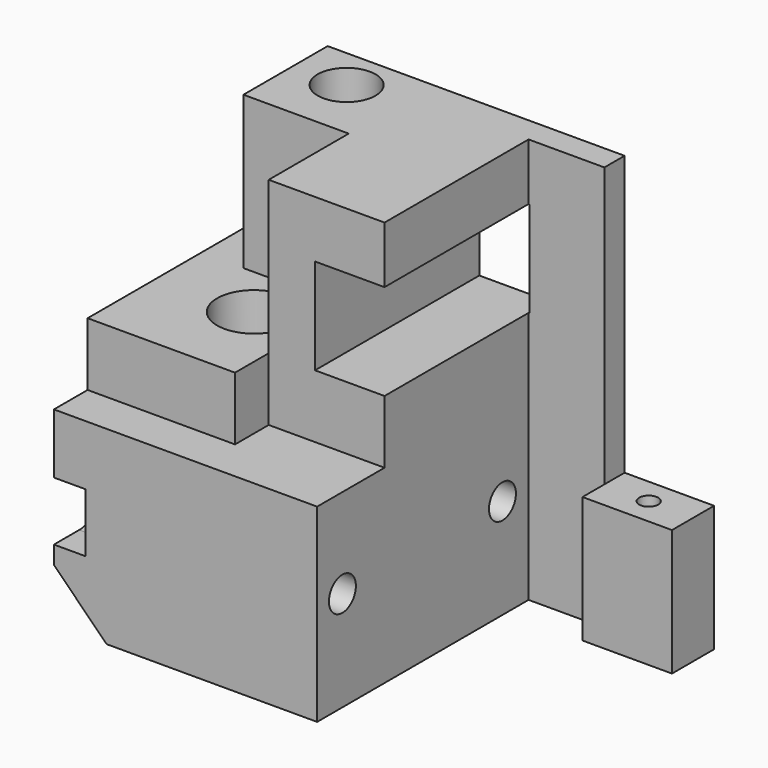
from build123d import *

# Parameters (mm, degrees)
F0_R          = 1.6
F1_DEPTH      = 16
F1_DEPTH_BACK = 9
F3_R          = 3.5
F3_R_2        = 1.4
F4_DEPTH      = 22
F5_DEPTH      = 16.501
F8_R          = 9.65
F9_DEPTH      = 5
F10_R         = 4.25
F11_DEPTH     = 6.5
F12_W         = 25
F12_H         = 9.1
F13_DEPTH     = 6.6
F14_R         = 2.8
F15_DEPTH     = 3
F16_W         = 8
F16_H         = 6
F16_H_2       = 9.1
F17_DEPTH     = 11
F23_W         = 8
F23_H         = 14.5
F24_DEPTH     = 25.001
F25_W         = 14
F25_H         = 9.5
F26_DEPTH     = 14.5
F28_DEPTH     = 9.0010001359
F29_W         = 14
F29_H         = 4
F30_DEPTH     = 6
F32_DEPTH     = 2.4
F33_W         = 10
F33_H         = 14.5
F34_DEPTH     = 4
F35_R         = 0.9
F36_DEPTH     = 3.2
F37_W         = 8.5
F37_H         = 12
F38_DEPTH     = 5
F39_R         = 0.9
F40_DEPTH     = 12
F41_SIZE      = 0.25
F42_T1_DEPTH  = 31.0668298797
F42_T3_DEPTH  = 28.5668298797


# Not quite as in the source:
# - a fillet or chamfer that OpenCascade refuses, or shapes differently, is made with other operations: its cross-section is extruded or revolved along the edge and cut away or added


with BuildPart() as f1:
    # F0 (on Right) → F1 (new body, two sides)
    with BuildSketch(Plane.YZ) as f1_sk:
        Polygon((-12.5, 0), (15, 0), (15, 38.5), (-10, 38.5), (-10, 24), (-12.5, 24), align=None)
        with Locations((-9.5, 9.5)):
            Circle(F0_R, mode=Mode.SUBTRACT)
        with Locations((9.5, 9.5)):
            Circle(F0_R, mode=Mode.SUBTRACT)
    extrude(amount=F1_DEPTH)
    extrude(f1_sk.sketch, amount=-F1_DEPTH_BACK)

    # F3 (on face) → F4 (cut)
    with BuildSketch(Plane(origin=(0, 0, 0), x_dir=(1, 0, 0), z_dir=(0, 0, -1))):
        Circle(F3_R)
        with Locations((-2.2609790798, 6.2119889676)):
            Circle(F3_R_2)
        with Locations((-4.2492507141, -5.0640598044)):
            Circle(F3_R_2)
        with Locations((6.5102297939, -1.1479291633)):
            Circle(F3_R_2)
    extrude(amount=-F4_DEPTH, mode=Mode.SUBTRACT)

    # F5 (cut, through all): a face of the model
    f5_faces = [f1.faces().sort_by_distance(p)[0] for p in [
        (0, 0, 22),
    ]]
    extrude(f5_faces, amount=-F5_DEPTH, mode=Mode.SUBTRACT)

    # F8 (on face) → F9 (cut)
    with BuildSketch(Plane(origin=(0, 0, 0), x_dir=(1, 0, 0), z_dir=(0, 0, -1))):
        Circle(F8_R)
    extrude(amount=-F9_DEPTH, mode=Mode.SUBTRACT)

    # F10 (on face) → F11 (cut)
    with BuildSketch(Plane(origin=(0, 0, 5), x_dir=(1, 0, 0), z_dir=(0, 0, -1))):
        Circle(F10_R)
    extrude(amount=-F11_DEPTH, mode=Mode.SUBTRACT)

    # F12 (on face) → F13 (cut)
    with BuildSketch(Plane.YZ.offset(16)):
        with Locations((2.5, 28.55)):
            Rectangle(F12_W, F12_H)
    extrude(amount=-F13_DEPTH, mode=Mode.SUBTRACT)

    # F14 (on face) → F15 (cut)
    with BuildSketch(Plane(origin=(-9, 0, 0), x_dir=(0, -1, 0), z_dir=(-1, 0, 0))):
        with Locations((-9.5, 9.5)):
            Circle(F14_R)
        with BuildLine():
            ThreePointArc((9.5, 6.7), (11.4798989873, 7.5201010127), (12.3, 9.5))
            ThreePointArc((12.3, 9.5), (11.4798989873, 11.4798989873), (9.5, 12.3))
            ThreePointArc((9.5, 12.3), (6.7, 9.5), (9.5, 6.7))
        make_face()
        with BuildLine():
            ThreePointArc((9.5, 12.3), (11.4798989873, 11.4798989873), (12.3, 9.5))
            ThreePointArc((12.3, 9.5), (11.4798989873, 7.5201010127), (9.5, 6.7))
            Line((9.5, 6.7), (12.5, 6.7))
            Line((12.5, 6.7), (12.5, 12.3))
            Line((12.5, 12.3), (9.5, 12.3))
        make_face()
    extrude(amount=-F15_DEPTH, mode=Mode.SUBTRACT)

    # F16 (on face) → F17 (cut)
    with BuildSketch(Plane.YZ.offset(16)):
        with Locations((-8.5, 21)):
            Rectangle(F16_W, F16_H)
        with Locations((-8.5, 28.55)):
            Rectangle(F16_W, F16_H_2)
    extrude(amount=-F17_DEPTH, mode=Mode.SUBTRACT)

    # F21 (on plane+point) → F22 (revolve, cut)
    with BuildSketch(Plane.XZ.offset(-11)):
        Polygon((0, 12.5), (0, 38.5), (-2.75, 38.5), (-2.75, 31.8), (-1.4, 31.8), (-1.4, 12.5), align=None)
    revolve(axis=Axis((0, 11, 25.5), (0, 0, 1)), mode=Mode.SUBTRACT)

    # F23 (on face) → F24 (cut, through all)
    with BuildSketch(Plane.YZ.offset(16)):
        with Locations((-8.5, 31.25)):
            Rectangle(F23_W, F23_H)
    extrude(amount=-F24_DEPTH, mode=Mode.SUBTRACT)

    # F25 (on face) → F26 (cut, through all)
    with BuildSketch(Plane.XY.offset(38.5)):
        with Locations((-2, 0.25)):
            Rectangle(F25_W, F25_H)
    extrude(amount=-F26_DEPTH, mode=Mode.SUBTRACT)

    # F27 (on face) → F28 (cut, through all)
    with BuildSketch(Plane(origin=(-9, 0, 0), x_dir=(0, -1, 0), z_dir=(-1, 0, 0))):
        with BuildLine():
            Line((-9.65, 0), (9.65, 0))
            ThreePointArc((9.65, 0), (7.4518594557, 3.5930041952), (3.4817380717, 5))
            Line((3.4817380717, 5), (-3.4817380717, 5))
            ThreePointArc((-3.4817380717, 5), (-7.4518594557, 3.5930041952), (-9.65, 0))
        make_face()
    extrude(amount=-F28_DEPTH, mode=Mode.SUBTRACT)

    # F29 (on face) → F30 (cut, through all)
    with BuildSketch(Plane.XY.offset(24)):
        with Locations((-2, -10.5)):
            Rectangle(F29_W, F29_H)
    extrude(amount=-F30_DEPTH, mode=Mode.SUBTRACT)

    # F31 (on face) → F32 (join)
    with BuildSketch(Plane(origin=(0, 15, 0), x_dir=(-1, 0, 0), z_dir=(0, 1, 0))):
        Polygon((-23.2, 0), (-16, 0), (-16, 24), (-16.1, 24), (-16.1, 33.1), (-16, 33.1), (-16, 38.5), (-23.2, 38.5), align=None)
    extrude(amount=-F32_DEPTH)

    # F33 (on face) → F34 (cut)
    with BuildSketch(Plane(origin=(-9, 0, 0), x_dir=(0, -1, 0), z_dir=(-1, 0, 0))):
        with Locations((-10, 31.25)):
            Rectangle(F33_W, F33_H)
    extrude(amount=-F34_DEPTH, mode=Mode.SUBTRACT)

    # F35 (on face) → F36 (cut)
    with BuildSketch(Plane(origin=(-5, 0, 0), x_dir=(0, -1, 0), z_dir=(-1, 0, 0))):
        with Locations((-10, 33.75)):
            Circle(F35_R)
        with Locations((-10, 27.25)):
            Circle(F35_R)
    extrude(amount=-F36_DEPTH, mode=Mode.SUBTRACT)

    # F37 (on face) → F38 (join)
    with BuildSketch(Plane(origin=(0, 15, 0), x_dir=(-1, 0, 0), z_dir=(0, 1, 0))):
        with Locations((-27.45, 6)):
            Rectangle(F37_W, F37_H)
    extrude(amount=-F38_DEPTH)

    # F39 (on face) → F40 (cut, through all)
    with BuildSketch(Plane.XY.offset(12)):
        with Locations((27.45, 12.55)):
            Circle(F39_R)
    extrude(amount=-F40_DEPTH, mode=Mode.SUBTRACT)

    # F41
    f41_edges = [f1.edges().sort_by_distance(p)[0] for p in [
        (-3.660979, -6.211989, 5),
        (5.11023, 1.147929, 5),
        (-5.649251, 5.06406, 5),
    ]]
    chamfer(f41_edges, length=F41_SIZE)

    # F42: chamfer of 5 on 2 edges, made by hand

    # F42_s2 → F42_t1 (cut)
    with BuildSketch(Plane.XZ.offset(-27.8584149398)):
        Polygon((-9, 5), (-4, 0), (-9, 0), align=None)
    extrude(amount=F42_T1_DEPTH, mode=Mode.SUBTRACT)

    # F42_s4 → F42_t3 (cut)
    with BuildSketch(Plane.XZ.offset(-3.2084149398)):
        Polygon((-9, 5), (-4, 0), (-9, 0), align=None)
    extrude(amount=F42_T3_DEPTH, mode=Mode.SUBTRACT)


solid = f1.part
